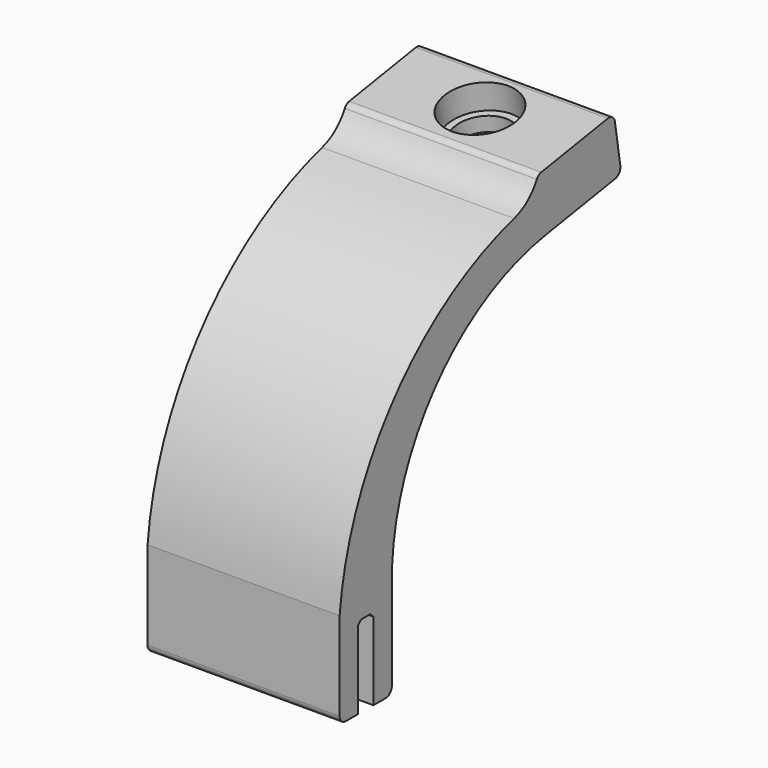
from build123d import *

# Parameters (mm, degrees)
F1_DEPTH       = 50
F2_DEPTH       = 5
F4_D           = 9.5
F4_CBORE_D     = 18.6
F4_CBORE_DEPTH = 7
F5_T1_DEPTH    = 50
F6_R           = 2
F7_R           = 2
F8_R           = 2
F9_R           = 2
F10_R          = 2
F11_SIZE       = 1
F12_SIZE       = 1
F3_R           = 7.4475
F3_R_2         = 4.7406141581
F13_DEPTH      = 11


# Not quite as in the source:
# - a fillet or chamfer that OpenCascade refuses, or shapes differently, is made with other operations: its cross-section is extruded or revolved along the edge and cut away or added
# - a feature names something its author has since deleted; it is built from what else it names


with BuildPart() as f1:
    # F0 (on Right) → F1 (new body)
    with BuildSketch(Plane.YZ):
        with BuildLine():
            Line((-36.8190155774, -18.3037728071), (-36.8190155774, -43.3037728071))
            Line((-36.8190155774, -43.3037728071), (-30.8190155774, -43.3037728071))
            Line((-30.8190155774, -43.3037728071), (-30.8190155774, -22.0011100173))
            Line((-30.8190155774, -22.0011100173), (-25.8190155774, -22.0011100173))
            Line((-25.8190155774, -22.0011100173), (-25.8190155774, -43.3037728071))
            Line((-25.8190155774, -43.3037728071), (-19.8190155774, -43.3037728071))
            Line((-19.8190155774, -43.3037728071), (-19.8190155774, -18.3037728071))
            ThreePointArc((-19.8190155774, -18.3037728071), (-6.0172669539, 21.0281033399), (30.1809844226, 41.6962271929))
            Line((30.1809844226, 41.6962271929), (54.8554914248, 45.7172599205))
            Line((54.8554914248, 45.7172599205), (53.2470783337, 55.5870627214))
            Line((53.2470783337, 55.5870627214), (28.5725713315, 51.5660299938))
            ThreePointArc((28.5725713315, 51.5660299938), (-16.0298177258, 27.7745861378), (-36.8190155774, -18.3037728071))
        make_face()
    extrude(amount=F1_DEPTH)

    # F2 (add): a face of the model
    f2_faces = [f1.faces().sort_by_distance(p)[0] for p in [
        (25, 40.9098248326, 53.5765463576),
    ]]
    extrude(f2_faces, amount=F2_DEPTH)

    # F4 (through all)
    with Locations(Plane(origin=(0, -8.2509991118, 50.6311062727), x_dir=(1, 0, 0), z_dir=(0, -0.1608413091, 0.9869802801))):
        with Locations((25, 48.9945122253)):
            CounterBoreHole(F4_D / 2, F4_CBORE_D / 2, F4_CBORE_DEPTH)

    # F5: fillet of radius 12 on 1 edges, made by hand

    # F5_s2 → F5_t1 (join)
    with BuildSketch(Plane.YZ):
        with BuildLine():
            ThreePointArc((19.9803220456, 49.6650925191), (24.650251765, 52.1990228082), (27.768364786, 56.5009313942))
            Line((27.768364786, 56.5009313942), (28.5725713315, 51.5660299938))
            ThreePointArc((28.5725713315, 51.5660299938), (24.2497369804, 50.7362893045), (19.9803220456, 49.6650925191))
        make_face()
    extrude(amount=F5_T1_DEPTH)

    # F6
    f6_edges = [f1.edges().sort_by_distance(p)[0] for p in [
        (25, 27.768365, 56.500931),
    ]]
    fillet(f6_edges, radius=F6_R)

    # F7
    f7_edges = [f1.edges().sort_by_distance(p)[0] for p in [
        (25, 52.442872, 60.521964),
    ]]
    fillet(f7_edges, radius=F7_R)

    # F8
    f8_edges = [f1.edges().sort_by_distance(p)[0] for p in [
        (25, 54.855491, 45.71726),
    ]]
    fillet(f8_edges, radius=F8_R)

    # F9
    f9_edges = [f1.edges().sort_by_distance(p)[0] for p in [
        (25, -19.819016, -43.303773),
    ]]
    fillet(f9_edges, radius=F9_R)

    # F10
    f10_edges = [f1.edges().sort_by_distance(p)[0] for p in [
        (25, -36.819016, -43.303773),
    ]]
    fillet(f10_edges, radius=F10_R)

    # F11
    f11_edges = [f1.edges().sort_by_distance(p)[0] for p in [
        (25, -30.819016, -22.00111),
    ]]
    chamfer(f11_edges, length=F11_SIZE)

    # F12
    f12_edges = [f1.edges().sort_by_distance(p)[0] for p in [
        (25, -25.819016, -22.00111),
    ]]
    chamfer(f12_edges, length=F12_SIZE)

    # F3 (on face) → F13 (cut)
    with BuildSketch(Plane(origin=(0, -8.2509991118, 50.6311062727), x_dir=(1, 0, 0), z_dir=(0, -0.1608413091, 0.9869802801))):
        with Locations((25, 48.9945122253)):
            Circle(F3_R)
        with Locations((25, 48.9945122253)):
            Circle(F3_R_2, mode=Mode.SUBTRACT)
    extrude(amount=-F13_DEPTH, mode=Mode.SUBTRACT)


solid = f1.part
